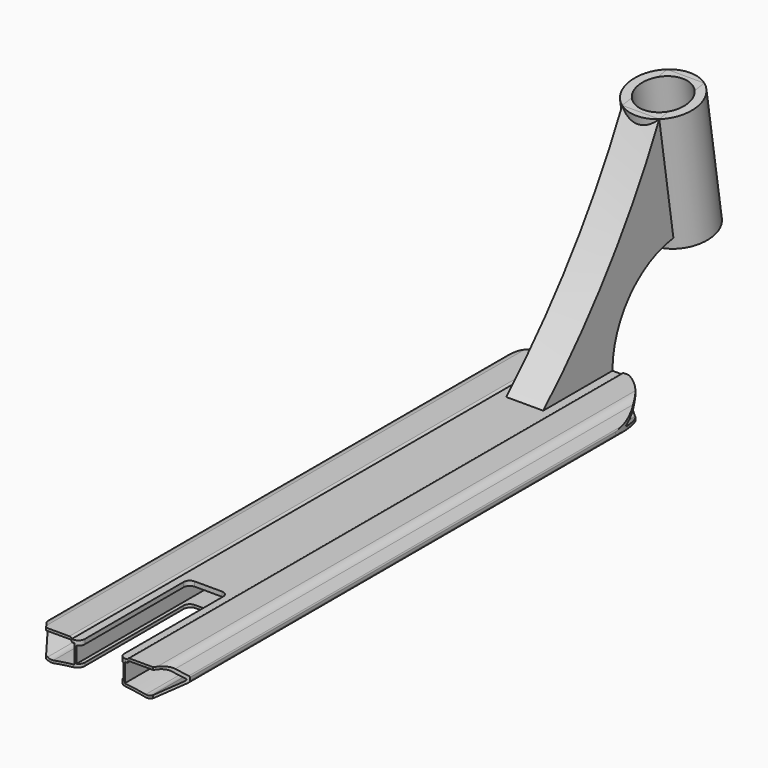
from build123d import *

# Parameters (mm, degrees)
F1_DEPTH       = 250
F2_W           = 38
F2_H           = 13
F3_DEPTH       = 250
F4_T1_DEPTH    = 509.3674969976
F5_R           = 9
F6_R           = 2
F8_DEPTH       = 764
F8_DEPTH_BACK  = 500.001
F10_DEPTH      = 22.2193051812
F10_DEPTH_BACK = 1.301
F12_DEPTH      = 1.3010001
F12_DEPTH_BACK = 22.219305294
F13_T1_DEPTH   = 3.7499991487
F13_T6_DEPTH   = 15.0134832828
F13_S7_R       = 200
F13_T8_DEPTH   = 10
F13_T12_DEPTH  = 15.0134832828
F13_S13_R      = 200
F13_T14_DEPTH  = 10
F13_T15_DEPTH  = 28.7499991487
F13_T17_DEPTH  = 27.5134832828
F15_DEPTH      = 15
F16_R          = 27.5
F17_DEPTH      = 100
F19_D          = 40


# Not quite as in the source:
# - a fillet or chamfer that OpenCascade refuses, or shapes differently, is made with other operations: its cross-section is extruded or revolved along the edge and cut away or added
# - an extrude ends at something that could not be found from the text; its depth is read off the source's solid


with BuildPart() as f1:
    # F0 (on Front) → F1 (new body, symmetric)
    with BuildSketch(Plane.XZ):
        with BuildLine():
            Line((22.5, 0), (0, 0))
            Line((0, 0), (-22.5, 0))
            Line((-22.5, 0), (-22.5, 1.3))
            Line((-22.5, 1.3), (-49.1090036882, 1.3))
            Line((-49.1090036882, 1.3), (-57.5, -8.7))
            Line((-57.5, -8.7), (-57.5, -12.7))
            Line((-57.5, -12.7), (-40.1794919243, -22.7))
            ThreePointArc((-40.1794919243, -22.7), (0, -18.6224551416), (40.1794919243, -22.7))
            Line((40.1794919243, -22.7), (57.5, -12.7))
            Line((57.5, -12.7), (57.5, -8.7))
            Line((57.5, -8.7), (49.1090036882, 1.3))
            Line((49.1090036882, 1.3), (22.5, 1.3))
            Line((22.5, 1.3), (22.5, 0))
        make_face()
    extrude(amount=F1_DEPTH, both=True)

    # F2 (on Front) → F3 (cut, symmetric)
    with BuildSketch(Plane.XZ):
        with Locations((0, -10.2499991487)):
            Rectangle(F2_W, F2_H)
    extrude(amount=F3_DEPTH, both=True, mode=Mode.SUBTRACT)

    # F4: fillet of radius 2 on 2 edges, made by hand

    # F4_s2 → F4_t1 (cut)
    with BuildSketch(Plane.XZ.offset(-254.6837484988)):
        with BuildLine():
            ThreePointArc((24.3734993995, 1.3), (23.2333239744, 0.9431676725), (22.5, 0))
            Line((22.5, 0), (22.5, 1.3))
            Line((22.5, 1.3), (24.3734993995, 1.3))
        make_face()
        with BuildLine():
            ThreePointArc((-24.3734993995, 1.3), (-23.2333239744, 0.9431676725), (-22.5, 0))
            Line((-22.5, 0), (-22.5, 1.3))
            Line((-22.5, 1.3), (-24.3734993995, 1.3))
        make_face()
    extrude(amount=F4_T1_DEPTH, mode=Mode.SUBTRACT)

    # F5
    f5_edges = [f1.edges().sort_by_distance(p)[0] for p in [
        (-49.109004, 0, 1.3),
        (49.109004, 0, 1.3),
        (40.179492, 0, -22.7),
        (-40.179492, 0, -22.7),
    ]]
    fillet(f5_edges, radius=F5_R)

    # F6
    f6_edges = [f1.edges().sort_by_distance(p)[0] for p in [
        (-57.5, 0, -8.7),
        (-57.5, 0, -12.7),
        (57.5, 0, -8.7),
        (57.5, 0, -12.7),
    ]]
    fillet(f6_edges, radius=F6_R)

    # F7 (on face) → F8 (cut, two sides)
    with BuildSketch(Plane.XZ.offset(250)) as f8_sk:
        with BuildLine():
            ThreePointArc((-37.3093701274, -20.0978700124), (-28.8776819579, -18.697270423), (-20.3942914958, -17.6546147432))
            Line((-20.3942914958, -17.6546147432), (-20.3942914958, -2.4123612095))
            Line((-20.3942914958, -2.4123612095), (-22.3942914958, -2.4123612095))
            ThreePointArc((-22.3942914958, -2.4123612095), (-23.0649271969, -1.1875057717), (-24.3734993995, -0.7))
            Line((-24.3734993995, -0.7), (-44.9122347648, -0.7))
            ThreePointArc((-44.9122347648, -0.7), (-47.870562597, -1.3558454907), (-50.2745458667, -3.2004867322))
            Line((-50.2745458667, -3.2004867322), (-55.9308095341, -9.9413592785))
            ThreePointArc((-55.9308095341, -9.9413592785), (-56.149572844, -10.7577950659), (-55.664765091, -11.450172292))
            Line((-55.664765091, -11.450172292), (-42.1022690923, -19.2804830077))
            ThreePointArc((-42.1022690923, -19.2804830077), (-39.7790673433, -20.1186780608), (-37.3093701274, -20.0978700124))
        make_face()
        with BuildLine():
            Line((22.3942914958, -2.4123612095), (20.3942914958, -2.4123612095))
            Line((20.3942914958, -2.4123612095), (20.3942914958, -17.6546147432))
            ThreePointArc((20.3942914958, -17.6546147432), (28.8776819579, -18.697270423), (37.3093701274, -20.0978700124))
            ThreePointArc((37.3093701274, -20.0978700124), (39.7790673433, -20.1186780608), (42.1022690923, -19.2804830077))
            Line((42.1022690923, -19.2804830077), (55.664765091, -11.450172292))
            ThreePointArc((55.664765091, -11.450172292), (56.149572844, -10.7577950659), (55.9308095341, -9.9413592785))
            Line((55.9308095341, -9.9413592785), (50.2745458667, -3.2004867322))
            ThreePointArc((50.2745458667, -3.2004867322), (47.870562597, -1.3558454907), (44.9122347648, -0.7))
            Line((44.9122347648, -0.7), (24.3734993995, -0.7))
            ThreePointArc((24.3734993995, -0.7), (23.0649271969, -1.1875057717), (22.3942914958, -2.4123612095))
        make_face()
    extrude(amount=F8_DEPTH, mode=Mode.SUBTRACT)
    extrude(f8_sk.sketch, amount=-F8_DEPTH_BACK, mode=Mode.SUBTRACT)

    # F9 (on Top) → F10 (cut, two sides)
    with BuildSketch(Plane.XY) as f10_sk:
        with BuildLine():
            ThreePointArc((-57.5, 200), (0, 257.5), (57.5, 200))
            Line((57.5, 200), (57.5, 280))
            Line((57.5, 280), (-57.5, 280))
            Line((-57.5, 280), (-57.5, 200))
        make_face()
    extrude(amount=-F10_DEPTH, mode=Mode.SUBTRACT)
    extrude(f10_sk.sketch, amount=F10_DEPTH_BACK, mode=Mode.SUBTRACT)

    # F11 (on Top) → F12 (cut, two sides)
    with BuildSketch(Plane.XY) as f12_sk:
        Polygon((-43.2975540478, -250), (-68, -216), (-68, -346), (68, -346), (68, -216), (43.2975540478, -250), (16, -250), (16, -140), (-16, -140), (-16, -250), align=None)
    extrude(amount=F12_DEPTH, mode=Mode.SUBTRACT)
    extrude(f12_sk.sketch, amount=-F12_DEPTH_BACK, mode=Mode.SUBTRACT)

    # F13: fillet of radius 5 on 8 edges, made by hand

    # F13_s2 → F13_t1 (join)
    with BuildSketch(Plane.XY.offset(-3.7499991487)):
        with BuildLine():
            ThreePointArc((-11, -140), (-14.5355339059, -141.4644660941), (-16, -145))
            Line((-16, -145), (-16, -140))
            Line((-16, -140), (-11, -140))
        make_face()
        with BuildLine():
            ThreePointArc((16, -145), (14.5355339059, -141.4644660941), (11, -140))
            Line((11, -140), (16, -140))
            Line((16, -140), (16, -145))
        make_face()
    extrude(amount=F13_T1_DEPTH)


with BuildPart() as f13_tool4:
    # F13_s5 → F13_t6 (new body)
    with BuildSketch(Plane.XY.offset(-16.7499991487)):
        with BuildLine():
            ThreePointArc((-16, -145), (-14.5355339059, -141.4644660941), (-11, -140))
            Line((-11, -140), (-16, -140))
            Line((-16, -140), (-16, -145))
        make_face()
    extrude(amount=-F13_T6_DEPTH)

    # F13_s7 → F13_t8 (cut, symmetric)
    with BuildSketch(Plane.XZ.offset(142.5)):
        with Locations((0, -218.6224551416)):
            Circle(F13_S7_R)
    extrude(amount=F13_T8_DEPTH, both=True, mode=Mode.SUBTRACT)


with BuildPart() as f1_1:
    add(f1.part)

    # F13_t3: union F13_tool4
    add(f13_tool4.part)


with BuildPart() as f13_tool10:
    # F13_s11 → F13_t12 (new body)
    with BuildSketch(Plane.XY.offset(-31.7634824315)):
        with BuildLine():
            ThreePointArc((16, -145), (14.5355339059, -141.4644660941), (11, -140))
            Line((11, -140), (16, -140))
            Line((16, -140), (16, -145))
        make_face()
    extrude(amount=F13_T12_DEPTH)

    # F13_s13 → F13_t14 (cut, symmetric)
    with BuildSketch(Plane.XZ.offset(142.5)):
        with Locations((0, -218.6224551416)):
            Circle(F13_S13_R)
    extrude(amount=F13_T14_DEPTH, both=True, mode=Mode.SUBTRACT)


with BuildPart() as f1_2:
    add(f1_1.part)

    # F13_t9: union F13_tool10
    add(f13_tool10.part)

    # F13_s16 → F13_t15 (cut)
    with BuildSketch(Plane.XY.offset(-16.2499991487)):
        with BuildLine():
            ThreePointArc((21, -250), (17.4644660941, -248.5355339059), (16, -245))
            Line((16, -245), (16, -250))
            Line((16, -250), (21, -250))
        make_face()
        with BuildLine():
            ThreePointArc((-21, -250), (-17.4644660941, -248.5355339059), (-16, -245))
            Line((-16, -245), (-16, -250))
            Line((-16, -250), (-21, -250))
        make_face()
    extrude(amount=F13_T15_DEPTH, mode=Mode.SUBTRACT)

    # F13_s18 → F13_t17 (cut)
    with BuildSketch(Plane.XY.offset(-31.7634824315)):
        with BuildLine():
            ThreePointArc((21, -250), (17.4644660941, -248.5355339059), (16, -245))
            Line((16, -245), (16, -250))
            Line((16, -250), (21, -250))
        make_face()
        with BuildLine():
            ThreePointArc((-21, -250), (-17.4644660941, -248.5355339059), (-16, -245))
            Line((-16, -245), (-16, -250))
            Line((-16, -250), (-21, -250))
        make_face()
    extrude(amount=F13_T17_DEPTH, mode=Mode.SUBTRACT)

    # F14 (on Right) → F15 (join, symmetric)
    with BuildSketch(Plane.YZ):
        with BuildLine():
            ThreePointArc((297.3819995028, 160), (245.9666940414, 74.662277853), (180, 0))
            Line((180, 0), (250, 0))
            ThreePointArc((250, 0), (267.6550746197, 46.4758946867), (311.7145367693, 69.5079211245))
            Line((311.7145367693, 69.5079211245), (313.0254460068, 61.2311659405))
            Line((313.0254460068, 61.2311659405), (358.4591096742, 68.4271513323))
            Line((358.4591096742, 68.4271513323), (342.8156631702, 167.1959853919))
            Line((342.8156631702, 167.1959853919), (297.3819995028, 160))
        make_face()
    extrude(amount=F15_DEPTH, both=True)

    # F16 (on face) → F17 (join, through all)
    with BuildSketch(Plane(origin=(0, -17.4439040266, 110.1364754698), x_dir=(1, 0, 0), z_dir=(0, -0.156434465, 0.9876883406))):
        with Locations((0, 341.7502480182)):
            Circle(F16_R)
    extrude(amount=-F17_DEPTH)

    # F19 (through all)
    with Locations(Plane(origin=(0, -17.4439040266, 110.1364754698), x_dir=(1, 0, 0), z_dir=(0, -0.156434465, 0.9876883406))):
        with Locations((0, 341.7502480182)):
            Hole(F19_D / 2)


solid = f1_2.part
